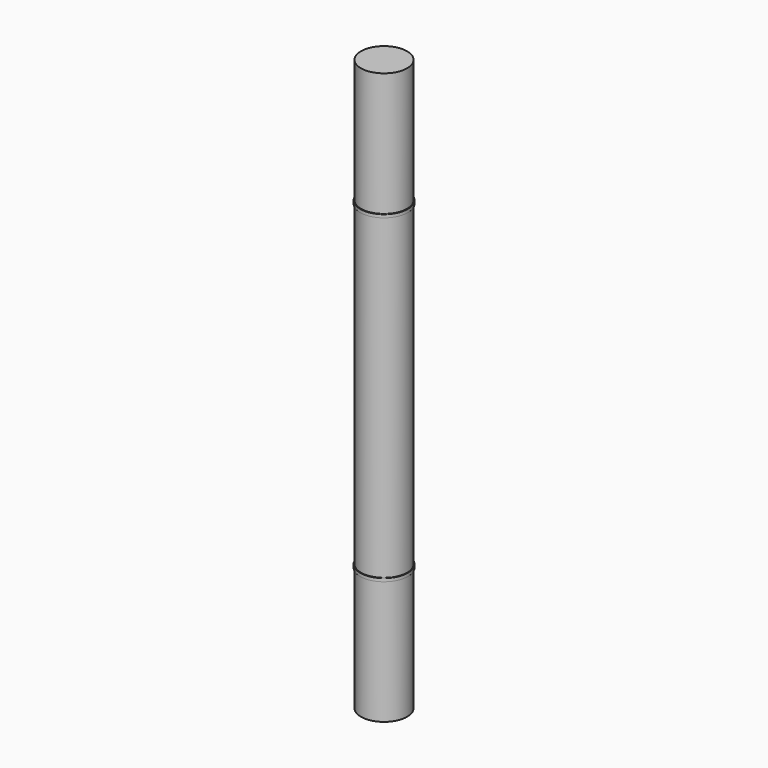
from build123d import *

# Parameters (mm, degrees)
F0_R          = 72.778
F1_DEPTH      = 900
F1_DEPTH_BACK = 900
F3_R          = 75
F3_R_2        = 72.778
F4_DEPTH      = 10


# Not quite as in the source:
# - a pattern or mirror of a feature is missing from the dataset's text; its kind, count and spacing are read off the source's solid


with BuildPart() as f1:
    # F0 (on Top) → F1 (new body, two sides)
    with BuildSketch(Plane.XY) as f1_sk:
        Circle(F0_R)
    extrude(amount=F1_DEPTH)
    extrude(f1_sk.sketch, amount=-F1_DEPTH_BACK)

    # F3 (on offset) → F4 (join)
    with BuildSketch(Plane.XY.offset(500)):
        Circle(F3_R)
        Circle(F3_R_2, mode=Mode.SUBTRACT)
    f4 = extrude(amount=F4_DEPTH)

    # F4_copies: F4 across plane
    add(f4.mirror(Plane(origin=(0, 0, 0), x_dir=(-1, 0, 0), z_dir=(0, 0, -1))))


solid = f1.part
